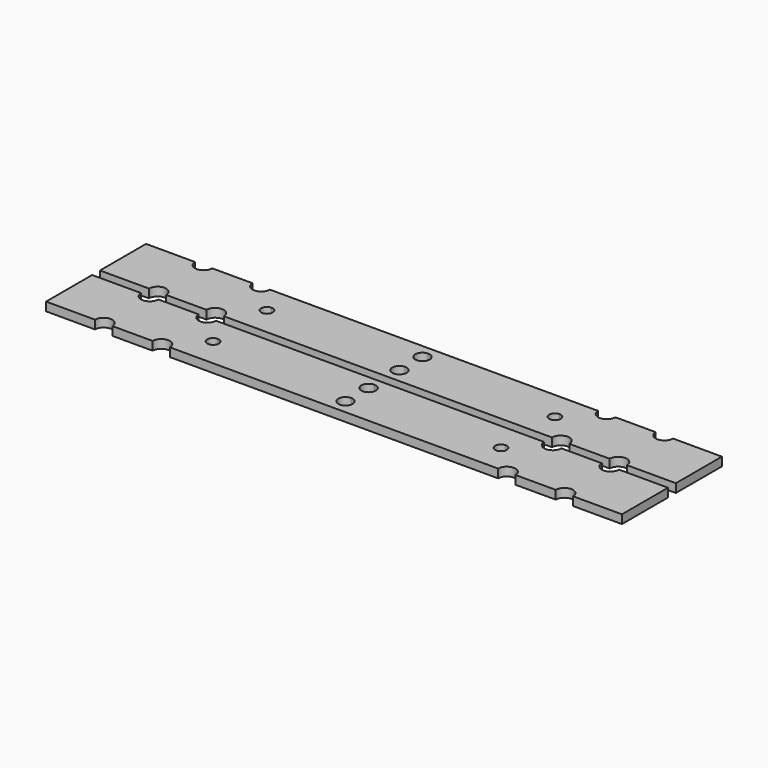
from build123d import *

# Parameters (mm, degrees)
F0_W     = 100
F0_H     = 20
F1_DEPTH = 1.5
F2_W     = 25
F2_H     = 5
F3_DEPTH = 1.501
F5_DEPTH = 1.501
F7_DEPTH = 1.501


with BuildPart() as f1:
    # F0 (on Top) → F1 (new body)
    with BuildSketch(Plane.XY):
        Rectangle(F0_W, F0_H)
    extrude(amount=F1_DEPTH)

    # F2 (on face) → F3 (cut, through all)
    with BuildSketch(Plane.XY.offset(1.5)):
        with BuildLine():
            Line((-25, -1), (-25, 1))
            ThreePointArc((-25, 1), (-26, 0), (-25, -1))
        make_face()
        with BuildLine():
            ThreePointArc((-24, 0), (-24.2928932188, 0.7071067812), (-25, 1))
            Line((-25, 1), (-25, -1))
            ThreePointArc((-25, -1), (-24.2928932188, -0.7071067812), (-24, 0))
        make_face()
        with BuildLine():
            Line((25, -1), (25, 1))
            ThreePointArc((25, 1), (24, 0), (25, -1))
        make_face()
        with BuildLine():
            ThreePointArc((26, 0), (25.7071067812, 0.7071067812), (25, 1))
            Line((25, 1), (25, -1))
            ThreePointArc((25, -1), (25.7071067812, -0.7071067812), (26, 0))
        make_face()
        with Locations((-37.5, 7.5)):
            Rectangle(F2_W, F2_H)
        with Locations((-12.5, 7.5)):
            Rectangle(F2_W, F2_H)
        with Locations((12.5, 7.5)):
            Rectangle(F2_W, F2_H)
        with Locations((37.5, 7.5)):
            Rectangle(F2_W, F2_H)
        with Locations((37.5, -7.5)):
            Rectangle(F2_W, F2_H)
        with Locations((12.5, -7.5)):
            Rectangle(F2_W, F2_H)
        with Locations((-12.5, -7.5)):
            Rectangle(F2_W, F2_H)
        with Locations((-37.5, -7.5)):
            Rectangle(F2_W, F2_H)
    extrude(amount=-F3_DEPTH, mode=Mode.SUBTRACT)

    # F4 (on face) → F5 (cut, through all)
    with BuildSketch(Plane.XY.offset(1.5)):
        with BuildLine():
            Line((-38.5, 5), (-41.5, 5))
            ThreePointArc((-41.5, 5), (-40, 3.5), (-38.5, 5))
        make_face()
        with BuildLine():
            ThreePointArc((-38.5, -5), (-40, -3.5), (-41.5, -5))
            Line((-41.5, -5), (-38.5, -5))
        make_face()
        with BuildLine():
            Line((-28.5, 5), (-31.5, 5))
            ThreePointArc((-31.5, 5), (-30, 3.5), (-28.5, 5))
        make_face()
        with BuildLine():
            ThreePointArc((-28.5, -5), (-30, -3.5), (-31.5, -5))
            Line((-31.5, -5), (-28.5, -5))
        make_face()
        with BuildLine():
            Line((31.5, 5), (28.5, 5))
            ThreePointArc((28.5, 5), (30, 3.5), (31.5, 5))
        make_face()
        with BuildLine():
            ThreePointArc((31.5, -5), (30, -3.5), (28.5, -5))
            Line((28.5, -5), (31.5, -5))
        make_face()
        with BuildLine():
            Line((41.5, 5), (38.5, 5))
            ThreePointArc((38.5, 5), (40, 3.5), (41.5, 5))
        make_face()
        with BuildLine():
            ThreePointArc((41.5, 5), (40, 6.5), (38.5, 5))
            Line((38.5, 5), (41.5, 5))
        make_face()
        with BuildLine():
            ThreePointArc((41.5, -5), (40, -3.5), (38.5, -5))
            Line((38.5, -5), (41.5, -5))
        make_face()
    extrude(amount=-F5_DEPTH, mode=Mode.SUBTRACT)

    # F6 (on face) → F7 (cut, through all)
    with BuildSketch(Plane.XY.offset(1.5)):
        with BuildLine():
            Line((0, 2.5), (0, 3.75))
            ThreePointArc((0, 3.75), (-1.25, 2.5), (0, 1.25))
            Line((0, 1.25), (0, 2.5))
        make_face()
        with BuildLine():
            ThreePointArc((1.25, 2.5), (0.8838834765, 3.3838834765), (0, 3.75))
            Line((0, 3.75), (0, 2.5))
            Line((0, 2.5), (0, 1.25))
            ThreePointArc((0, 1.25), (0.8838834765, 1.6161165235), (1.25, 2.5))
        make_face()
        with BuildLine():
            ThreePointArc((1.25, -2.5), (0.8838834765, -1.6161165235), (0, -1.25))
            Line((0, -1.25), (0, -2.5))
            Line((0, -2.5), (0, -3.75))
            ThreePointArc((0, -3.75), (0.8838834765, -3.3838834765), (1.25, -2.5))
        make_face()
        with BuildLine():
            Line((0, -2.5), (0, -1.25))
            ThreePointArc((0, -1.25), (-1.25, -2.5), (0, -3.75))
            Line((0, -3.75), (0, -2.5))
        make_face()
    extrude(amount=-F7_DEPTH, mode=Mode.SUBTRACT)


with BuildPart() as f8_1:
    # F8: copy of F1
    add(f1.part.moved(Location((0, -11.7, 0))))


solid = Compound([f1.part, f8_1.part])
